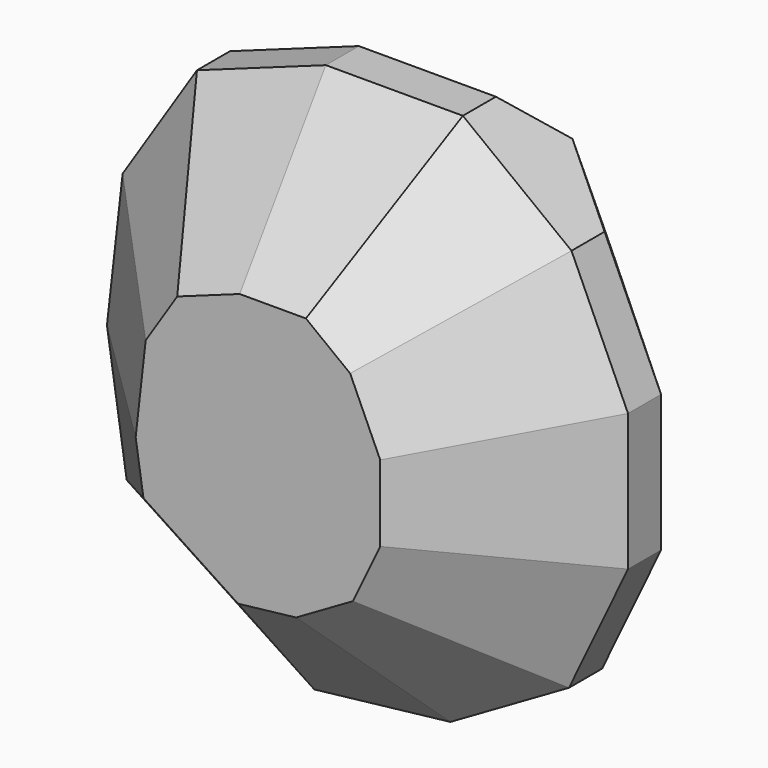
from build123d import *

# Parameters (mm, degrees)
F1_DEPTH     = 76.2
F2_SIZE      = 25.4
F3_T1_DEPTH  = 325.0997163693
F3_T3_DEPTH  = 325.0997163693
F3_T5_DEPTH  = 247.368026375
F3_T7_DEPTH  = 325.557153853
F3_T9_DEPTH  = 263.50961712
F3_T11_DEPTH = 247.368026375
F3_T13_DEPTH = 247.368026375
F3_T15_DEPTH = 247.368026375
F3_T17_DEPTH = 247.368026375
F3_T19_DEPTH = 247.368026375
F3_T24_DEPTH = 324.0493372034
F3_T29_DEPTH = 324.0493372034
F3_T34_DEPTH = 247.368026375
F3_T39_DEPTH = 247.368026375


# Not quite as in the source:
# - a fillet or chamfer that OpenCascade refuses, or shapes differently, is made with other operations: its cross-section is extruded or revolved along the edge and cut away or added


with BuildPart() as f1:
    # F0 (on Front) → F1 (new body)
    with BuildSketch(Plane.XZ):
        Polygon((-22.9806532577, 64.0975162387), (-46.7637702823, 55.5351264775), (-60.4687564512, 34.2954342025), (-63.3636489511, 8.723853156), (-59.7226433456, -15.2280917391), (-25.1116699455, -37.9793605928), (0, -35.0888232076), (21.8782797456, -22.4281735718), (32.7606478844, 0.3868486179), (32.7606478844, 25.6643321522), (22.3381376327, 48.6930632045), (2.2968302766, 64.0975162387), align=None)
    extrude(amount=F1_DEPTH)

    # F2
    f2_edges = [f1.edges().sort_by_distance(p)[0] for p in [
        (-61.543146, -76.2, -3.252119),
        (-42.417157, -76.2, -26.603726),
        (-12.555835, -76.2, -36.534092),
        (10.93914, -76.2, -28.758498),
        (27.319464, -76.2, -11.020662),
        (32.760648, -76.2, 13.02559),
        (27.549393, -76.2, 37.178698),
        (12.317484, -76.2, 56.39529),
        (-10.341911, -76.2, 64.097516),
        (-34.872212, -76.2, 59.816321),
        (-53.616263, -76.2, 44.91528),
        (-61.916203, -76.2, 21.509644),
    ]]
    chamfer(f2_edges, length=F2_SIZE)

    # F3: chamfer of 43.18 on 12 edges, made by hand

    # F3_s2 → F3_t1 (cut)
    with BuildSketch(Plane.YZ.offset(-211.7576146723)):
        Polygon((-43.18, 64.0975162387), (0, 20.9175162387), (0, 64.0975162387), align=None)
    extrude(amount=F3_T1_DEPTH, mode=Mode.SUBTRACT)

    # F3_s4 → F3_t3 (cut)
    with BuildSketch(Plane(origin=(177.7014842233, 0, 63.9760283522), x_dir=(0, 1, 0), z_dir=(-0.9408815158, 0, -0.3387358457))):
        Polygon((0, -24.9125392558), (-43.18, -68.0925392558), (0, -68.0925392558), align=None)
    extrude(amount=F3_T3_DEPTH, mode=Mode.SUBTRACT)

    # F3_s6 → F3_t5 (cut)
    with BuildSketch(Plane(origin=(71.76035528, 0, 111.212652454), x_dir=(0, 1, 0), z_dir=(-0.5421815882, 0, -0.8402613435))):
        Polygon((0, -26.2239115206), (-43.18, -69.4039115206), (0, -69.4039115206), align=None)
    extrude(amount=F3_T5_DEPTH, mode=Mode.SUBTRACT)

    # F3_s8 → F3_t7 (cut)
    with BuildSketch(Plane(origin=(15.5595712054, 0, 137.4430436178), x_dir=(0, 1, 0), z_dir=(-0.1124888822, 0, -0.9936529834))):
        Polygon((0, -20.7628153082), (-43.18, -63.9428153082), (0, -63.9428153082), align=None)
    extrude(amount=F3_T7_DEPTH, mode=Mode.SUBTRACT)

    # F3_s10 → F3_t9 (cut)
    with BuildSketch(Plane(origin=(-127.5057052722, 0, 83.8149377508), x_dir=(0, 1, 0), z_dir=(0.8356288498, 0, -0.5492944796))):
        Polygon((0, -2.3503510843), (-43.18, -45.5303510843), (0, -45.5303510843), align=None)
    extrude(amount=F3_T9_DEPTH, mode=Mode.SUBTRACT)

    # F3_s12 → F3_t11 (cut)
    with BuildSketch(Plane(origin=(-139.4146792436, 0, -16.0476520785), x_dir=(0, 1, 0), z_dir=(0.9934402652, 0, 0.1143522606))):
        Polygon((0, 8.3213501676), (-43.18, -34.8586498324), (0, -34.8586498324), align=None)
    extrude(amount=F3_T11_DEPTH, mode=Mode.SUBTRACT)

    # F3_s14 → F3_t13 (cut)
    with BuildSketch(Plane(origin=(-111.323834941, 0, -64.4215215589), x_dir=(0, 1, 0), z_dir=(0.8655244386, 0, 0.500866695))):
        Polygon((0, 12.8097659916), (-43.18, -30.3702340084), (0, -30.3702340084), align=None)
    extrude(amount=F3_T13_DEPTH, mode=Mode.SUBTRACT)

    # F3_s16 → F3_t15 (cut)
    with BuildSketch(Plane(origin=(-52.4668465727, 0, -109.9974062184), x_dir=(0, 1, 0), z_dir=(0.4305162784, 0, 0.9025828128))):
        Polygon((0, 13.7773469096), (-43.18, -29.4026530904), (0, -29.4026530904), align=None)
    extrude(amount=F3_T15_DEPTH, mode=Mode.SUBTRACT)

    # F3_s18 → F3_t17 (cut)
    with BuildSketch(Plane.XY.offset(-110.6584228025)):
        Polygon((-10.4193521156, 0), (32.7606478844, -43.18), (32.7606478844, 0), align=None)
    extrude(amount=F3_T17_DEPTH, mode=Mode.SUBTRACT)

    # F3_s20 → F3_t19 (cut)
    with BuildSketch(Plane(origin=(41.7156753309, 0, -92.1715637275), x_dir=(0, 1, 0), z_dir=(-0.4123238865, 0, 0.9110373278))):
        Polygon((0, 2.7518097175), (-43.18, -40.4281902825), (0, -40.4281902825), align=None)
    extrude(amount=F3_T19_DEPTH, mode=Mode.SUBTRACT)


with BuildPart() as f3_tool22:
    # F3_s23 → F3_t24 (new body)
    with BuildSketch(Plane(origin=(-31.0979390453, 0, 204.5742860839), x_dir=(0, 1, 0), z_dir=(0.150286454, 0, -0.9886424944))):
        Polygon((0, -18.1529189981), (-43.18, -61.3329189981), (0, -61.3329189981), align=None)
    extrude(amount=F3_T24_DEPTH)

    split(bisect_by=Plane(origin=(-10.3155166871, 10.3814076541, 1.1677929431), x_dir=(-0.7093543397, -0.7048520559, 0), z_dir=(-0.7026187627, 0.7071067812, 0.0795416514)), keep=Keep.TOP)


with BuildPart() as f1_1:
    add(f1.part)

    # F3_t21: cut F3_tool22
    add(f3_tool22.part, mode=Mode.SUBTRACT)


with BuildPart() as f3_tool27:
    # F3_s28 → F3_t29 (new body)
    with BuildSketch(Plane(origin=(-31.0979390453, 0, 204.5742860839), x_dir=(0, 1, 0), z_dir=(0.150286454, 0, -0.9886424944))):
        Polygon((0, -18.1529189981), (-43.18, -61.3329189981), (0, -61.3329189981), align=None)
    extrude(amount=F3_T29_DEPTH)

    split(bisect_by=Plane(origin=(-0.6455174379, 1.1751755422, -0.9820105866), x_dir=(-0.876476897, -0.481443921, 0), z_dir=(-0.3884098514, 0.7071067812, -0.5908788263)), keep=Keep.TOP)


with BuildPart() as f1_2:
    add(f1_1.part)

    # F3_t26: cut F3_tool27
    add(f3_tool27.part, mode=Mode.SUBTRACT)


with BuildPart() as f3_tool32:
    # F3_s33 → F3_t34 (new body)
    with BuildSketch(Plane(origin=(78.5572793932, 0, -60.3818852432), x_dir=(0, 1, 0), z_dir=(-0.7928521575, 0, 0.609414027))):
        Polygon((-43.18, -52.2195746281), (0, -9.0395746281), (0, -52.2195746281), align=None)
    extrude(amount=F3_T34_DEPTH)

    split(bisect_by=Plane(origin=(-1.2535006858, -1.3759048587, -0.5673184388), x_dir=(-0.7392234901, 0.6734601931, 0), z_dir=(0.6442006724, 0.7071067812, 0.2915570162)), keep=Keep.TOP)


with BuildPart() as f1_3:
    add(f1_2.part)

    # F3_t31: cut F3_tool32
    add(f3_tool32.part, mode=Mode.SUBTRACT)


with BuildPart() as f3_tool37:
    # F3_s38 → F3_t39 (new body)
    with BuildSketch(Plane(origin=(78.5572793932, 0, -60.3818852432), x_dir=(0, 1, 0), z_dir=(-0.7928521575, 0, 0.609414027))):
        Polygon((-43.18, -52.2195746281), (0, -9.0395746281), (0, -52.2195746281), align=None)
    extrude(amount=F3_T39_DEPTH)

    split(bisect_by=Plane(origin=(0, 10.4587581193, 10.4587581193), x_dir=(1, 0, 0), z_dir=(0, 0.7071067812, 0.7071067812)), keep=Keep.TOP)


with BuildPart() as f1_4:
    add(f1_3.part)

    # F3_t36: cut F3_tool37
    add(f3_tool37.part, mode=Mode.SUBTRACT)


solid = f1_4.part
